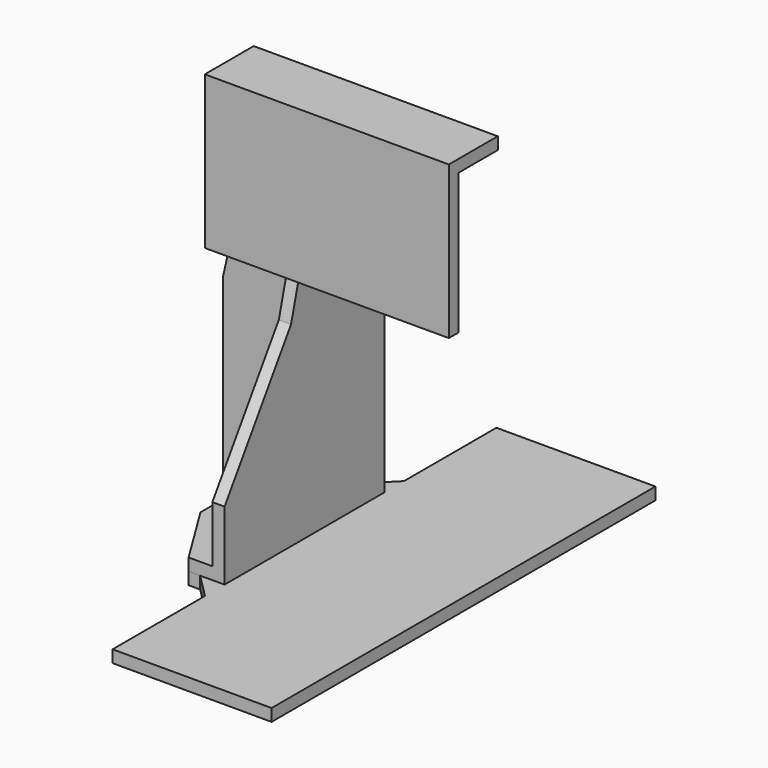
from build123d import *

# Parameters (mm, degrees)
F1_DEPTH      = 12.7
F3_DEPTH      = 12.7
F5_DEPTH      = 6.35
F5_DEPTH_BACK = 6.35
F7_DEPTH      = 25.4
F8_START      = 177.8
F8_DEPTH      = 12.7
F10_DEPTH     = 12.7
F12_DEPTH     = 12.7
F13_SIZE      = 25.4
F14_W         = 253.4000277519
F14_H         = 146.0330784321
F15_DEPTH     = 12.7
F16_W         = 12.7
F16_H         = 146.0330784321
F17_DEPTH     = 50.8
F18_W         = 253.4000277519
F18_H         = 63.5
F19_DEPTH     = 12.7


with BuildPart() as f1:
    # F0 (on Top) → F1 (new body)
    with BuildSketch(Plane.XY):
        Polygon((-244.4749832617, 35.8069409784), (-244.4749832617, 0), (-244.4749832617, -35.8069409784), (-202.4944386959, -103.7166595656), (-177.8, -103.7166595656), (-177.8, 0), (-177.8, 103.7166595656), (-202.4944386959, 103.7166595656), align=None)
    extrude(amount=F1_DEPTH)

    # F2 (on face) → F3 (join)
    with BuildSketch(Plane.YZ.offset(-177.8)):
        Polygon((-103.7166595656, 216.7370766401), (-103.7166595656, 0), (0, 0), (0, 390.6428515911), (-51.0313883424, 390.6428515911), align=None)
        Polygon((0, 390.6428515911), (0, 0), (103.7166595656, 0), (103.7166595656, 216.7370766401), (51.0313883424, 390.6428515911), align=None)
    extrude(amount=F3_DEPTH)

    # F4 (on Front) → F5 (join, two sides)
    with BuildSketch(Plane.XZ) as f5_sk:
        Polygon((-202.4944386959, 12.7), (-177.8, 12.7), (-177.8, 216.7370766401), (-177.8, 390.6428515911), (-205.6709676981, 390.6428515911), (-244.4749832617, 216.7370766401), (-244.4749832617, 12.7), align=None)
    extrude(amount=F5_DEPTH)
    extrude(f5_sk.sketch, amount=-F5_DEPTH_BACK)

    # F6 (on face) → F7 (cut)
    with BuildSketch(Plane(origin=(-177.8, 0, 0), x_dir=(0, -1, 0), z_dir=(-1, 0, 0))):
        Polygon((51.0313883424, 390.6428515911), (6.35, 390.6428515911), (6.35, 244.609773159), (17.4792539328, 202.7855962515), (84.4946950674, 216.7370766401), (103.7166595656, 216.7370766401), align=None)
        Polygon((84.4946950674, 216.7370766401), (17.4792539328, 202.7855962515), (103.7166595656, 71.3086128235), (103.7166595656, 216.7370766401), align=None)
    extrude(amount=-F7_DEPTH, mode=Mode.SUBTRACT)

    # F5_face1 (on face) → F8 (join)
    with BuildSketch(Plane(origin=(-205.6951011652, 47.7051250828, 12.7), x_dir=(1, 0, 0), z_dir=(0, 0, 1)).offset(F8_START)):
        Polygon((-38.7798820965, -11.8981841043), (-38.7798820965, -41.3551250828), (27.8951011652, -41.3551250828), (27.8951011652, 56.0115344828), (3.2006624693, 56.0115344828), align=None)
    extrude(amount=F8_DEPTH)

    # F9 (on face) → F10 (join)
    with BuildSketch(Plane.XY.offset(390.6428515911)):
        Polygon((-177.8, 6.35), (-177.8, 51.0313883424), (-205.6709676981, 6.35), align=None)
    extrude(amount=-F10_DEPTH)


with BuildPart() as f12:
    # F11 (on face) → F12 (new body)
    with BuildSketch(Plane(origin=(0, 0, 0), x_dir=(1, 0, 0), z_dir=(0, 0, -1))):
        Polygon((-165.1, -103.7166595656), (-165.1, 103.7166595656), (-202.4944386959, 103.7166595656), (-244.4749832617, 35.8069409784), (-244.4749832617, -35.8069409784), (-202.4944386959, -103.7166595656), align=None)
        Polygon((-165.1, 249.0800619125), (-165.1, 103.7166595656), (-165.1, -103.7166595656), (-165.1, -249.0800619125), (0, -249.0800619125), (0, 249.0800619125), align=None)
    extrude(amount=F12_DEPTH)

    # F13
    f13_edges = [f12.edges().sort_by_distance(p)[0] for p in [
        (-165.1, -103.71666, -6.35),
        (-165.1, 103.71666, -6.35),
    ]]
    chamfer(f13_edges, length=F13_SIZE)


with BuildPart() as f15:
    # F14 (on face) → F15 (new body)
    with BuildSketch(Plane.XZ.offset(6.35)):
        with Locations((-126.700013876, 317.6263123751)):
            Rectangle(F14_W, F14_H)
    extrude(amount=F15_DEPTH)

    # F16 (on face) → F17 (join)
    with BuildSketch(Plane(origin=(0, -6.35, 0), x_dir=(-1, 0, 0), z_dir=(0, 1, 0))):
        with Locations((158.75, 317.6263123751)):
            Rectangle(F16_W, F16_H)
    extrude(amount=F17_DEPTH)

    # F18 (on face) → F19 (join)
    with BuildSketch(Plane.XY.offset(390.6428515911)):
        with Locations((-126.700013876, 12.7)):
            Rectangle(F18_W, F18_H)
    extrude(amount=F19_DEPTH)


solid = Compound([f1.part, f12.part, f15.part])
